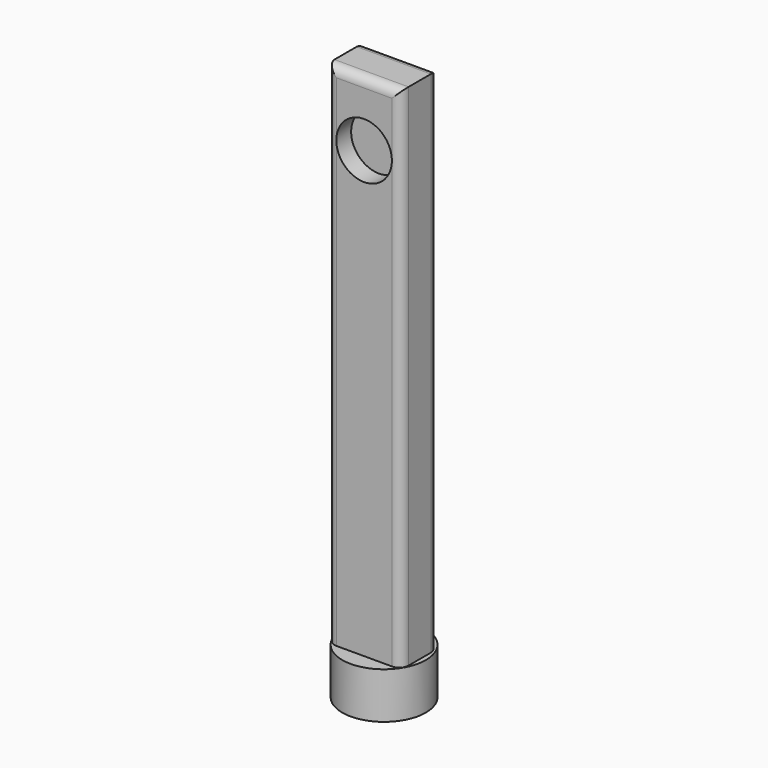
from build123d import *

# Parameters (mm, degrees)
F0_W     = 40
F0_H     = 300
F1_DEPTH = 25
F2_R     = 15
F3_DEPTH = 10
F4_R     = 5
F5_R     = 4.99999
F6_R     = 22.5487204306
F7_DEPTH = 25


# Not quite as in the source:
# - a fillet or chamfer is up to 0.001 mm smaller than in the source, because OpenCascade refuses the exact size


with BuildPart() as f1:
    # F0 (on Front) → F1 (new body)
    with BuildSketch(Plane.XZ):
        with Locations((0, 32.5)):
            Rectangle(F0_W, F0_H)
    extrude(amount=-F1_DEPTH)

    # F2 (on Front) → F3 (cut)
    with BuildSketch(Plane.XZ):
        with Locations((0, 147.7966460525)):
            Circle(F2_R)
    extrude(amount=-F3_DEPTH, mode=Mode.SUBTRACT)

    # F4
    f4_edges = [f1.edges().sort_by_distance(p)[0] for p in [
        (20, 25, 32.5),
        (-20, 25, 32.5),
        (0, 25, 182.5),
    ]]
    fillet(f4_edges, radius=F4_R)

    # F5 (radius 5 in the source; OpenCascade refuses exactly that, so slightly less here)
    f5_edges = [f1.edges().sort_by_distance(p)[0] for p in [
        (20, 0, 32.5),
        (-20, 0, 32.5),
        (0, 0, 182.5),
    ]]
    fillet(f5_edges, radius=F5_R)

    # F6 (on face) → F7 (join)
    with BuildSketch(Plane(origin=(0, 0, -117.5), x_dir=(1, 0, 0), z_dir=(0, 0, -1))):
        with Locations((0, -13.4554868564)):
            Circle(F6_R)
    extrude(amount=-F7_DEPTH)


solid = f1.part
